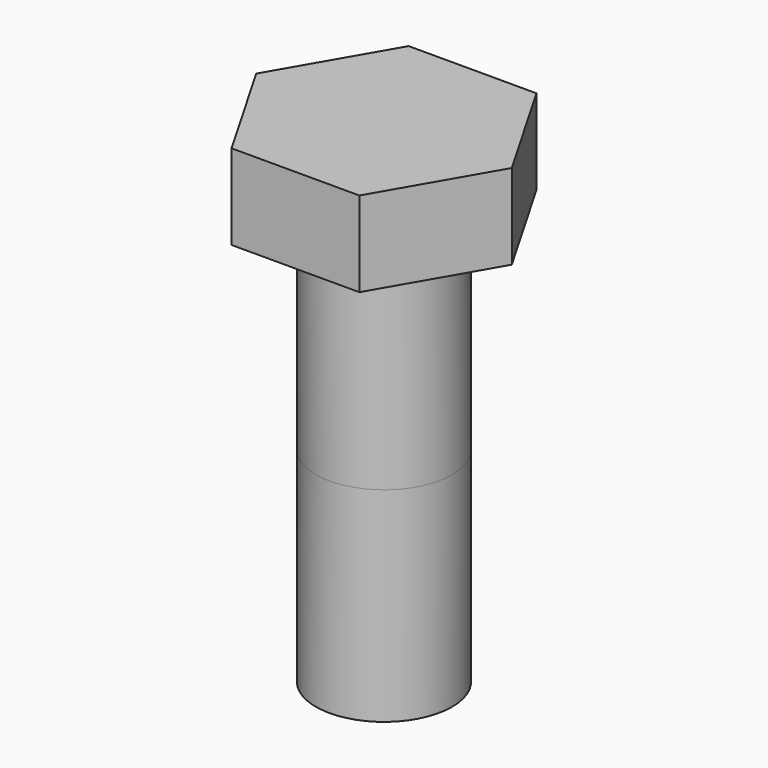
from build123d import *

# Parameters (mm, degrees)
F0_R          = 12.7
F1_DEPTH      = 38.1
F1_DEPTH_BACK = 38.1
F3_DEPTH      = 15.875


# Not quite as in the source:
# - a feature names something its author has since deleted; it is built from what else it names


with BuildPart() as f1:
    # F0 (on Top) → F1 (new body, two sides)
    with BuildSketch(Plane.XY) as f1_sk:
        Circle(F0_R)
    extrude(amount=-F1_DEPTH)
    extrude(f1_sk.sketch, amount=F1_DEPTH_BACK)

    # F2 (on face) → F3 (join)
    with BuildSketch(Plane.XY.offset(38.1)):
        Polygon((11.9150661804, 20.6375), (-11.9150661804, 20.6375), (-23.8301323608, 0), (-11.9150661804, -20.6375), (11.9150661804, -20.6375), (23.8301323608, 0), align=None)
    extrude(amount=F3_DEPTH)


solid = f1.part
